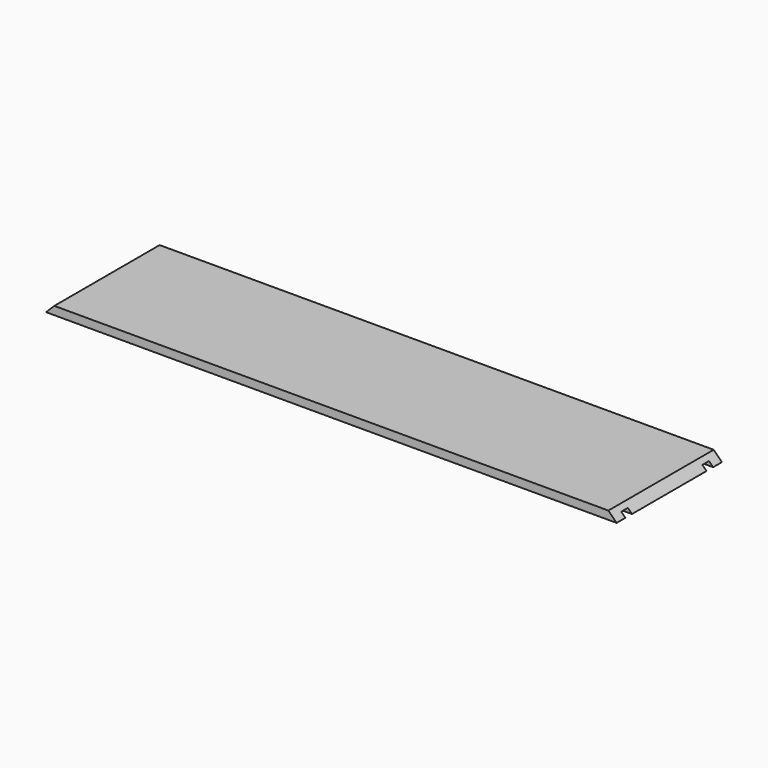
from build123d import *

# Parameters (mm, degrees)
F0_W     = 1320.8
F0_H     = 304.8
F1_DEPTH = 19.05
F2_SIZE  = 19.04999
F3_W     = 1320.8
F3_H     = 19.05
F4_DEPTH = 9.525


# Not quite as in the source:
# - a fillet or chamfer is up to 0.001 mm smaller than in the source, because OpenCascade refuses the exact size


with BuildPart() as f1:
    # F0 (on Top) → F1 (new body)
    with BuildSketch(Plane.XY):
        with Locations((47.3523183346, -92.4993205261)):
            Rectangle(F0_W, F0_H)
    extrude(amount=F1_DEPTH)

    # F2 (size 19.05 in the source; OpenCascade refuses exactly that, so slightly less here)
    f2_edges = [f1.edges().sort_by_distance(p)[0] for p in [
        (707.752318, -92.499321, 19.05),
        (-613.047682, -92.499321, 19.05),
    ]]
    chamfer(f2_edges, length=F2_SIZE)

    # F3 (on face) → F4 (cut)
    with BuildSketch(Plane(origin=(0, 0, 0), x_dir=(1, 0, 0), z_dir=(0, 0, -1))):
        with Locations((47.3523183346, 209.9743205261)):
            Rectangle(F3_W, F3_H)
        with Locations((47.3523183346, -24.9756794739)):
            Rectangle(F3_W, F3_H)
    extrude(amount=-F4_DEPTH, mode=Mode.SUBTRACT)


solid = f1.part
